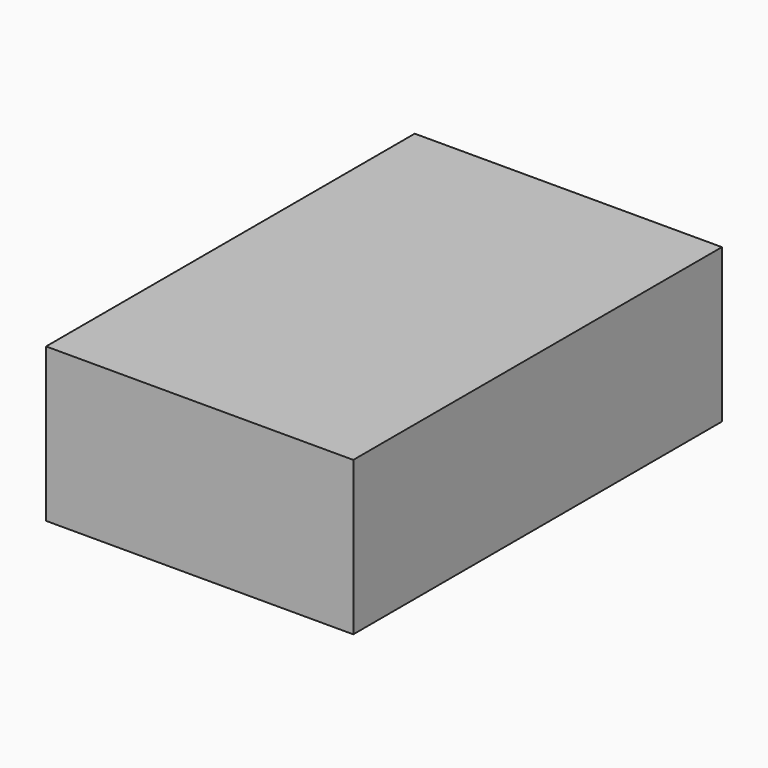
from build123d import *

# Parameters (mm, degrees)
F0_W     = 50.8
F0_H     = 25.4
F1_DEPTH = 76.2


# Not quite as in the source:
# - the program builds the solid bodies; features that only make, move or delete a surface that nothing else refers to are left out


with BuildPart() as f1:
    # F0 (on Front) → F1 (new body)
    with BuildSketch(Plane.XZ):
        with Locations((25.4, 12.7)):
            Rectangle(F0_W, F0_H)
    extrude(amount=F1_DEPTH)


solid = f1.part
